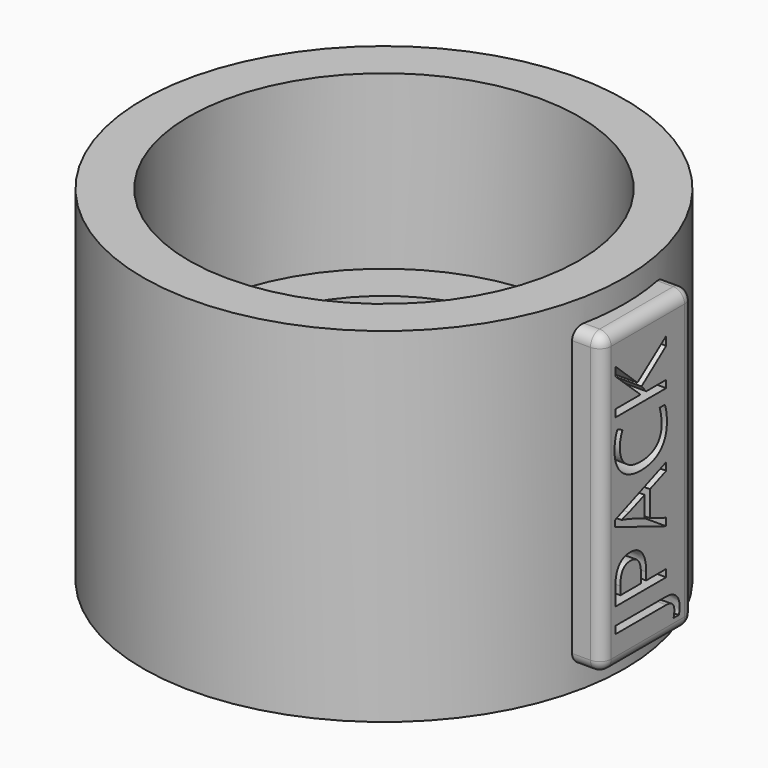
from build123d import *

# Parameters (mm, degrees)
F3_R          = 10.5
F4_DEPTH      = 2
F0_R          = 10.5
F0_R_2        = 6.5
F5_DEPTH      = 5.5
F6_R          = 10.5
F6_R_2        = 8.5
F7_DEPTH      = 7.5
F10_DEPTH     = 2
F11_R         = 0.5
F12_TEXT_SIZE = 3.8888888889
F13_DEPTH     = 5
F14_DEPTH     = 25


# Not quite as in the source:
# - Text() gives the source's letters only with a copy of the font that has no kerning and outlines rounded to 1/6400 em; it was checked with that copy


with BuildPart() as f4:
    # F3 (on offset) → F4 (new body)
    with BuildSketch(Plane.XY.offset(5.5)):
        Circle(F3_R)
    extrude(amount=F4_DEPTH)

    # F0 (on Top) → F5 (join)
    with BuildSketch(Plane.XY):
        Circle(F0_R)
        Circle(F0_R_2, mode=Mode.SUBTRACT)
    extrude(amount=F5_DEPTH)

    # F6 (on offset) → F7 (join)
    with BuildSketch(Plane.XY.offset(7.5)):
        Circle(F6_R)
        Circle(F6_R_2, mode=Mode.SUBTRACT)
    extrude(amount=F7_DEPTH)

    # F9 (on offset) → F10 (join)
    with BuildSketch(Plane.YZ.offset(9.5)):
        Polygon((-2.5, 1), (0, 1), (2.5, 1), (2.5, 14), (0, 14), (-2.5, 14), align=None)
    extrude(amount=F10_DEPTH)

    # F11
    f11_edges = [f4.edges().sort_by_distance(p)[0] for p in [
        (11.5, 0, 14),
        (11.5, 2.5, 7.5),
        (11.5, 0, 1),
        (11.5, -2.5, 7.5),
        (10.84902, 2.5, 14),
        (10.84902, 2.5, 1),
        (10.84902, -2.5, 14),
        (10.84902, -2.5, 1),
    ]]
    fillet(f11_edges, radius=F11_R)

    # F12 (on offset) → F13 (cut)
    with BuildSketch(Plane.YZ.offset(9.5)):
        with Locations(Location((1, 2), (0, 0, 90))):
            Text('JPACK', F12_TEXT_SIZE, font='Open Sans', text_align=(TextAlign.LEFT, TextAlign.BOTTOM))
    extrude(amount=F13_DEPTH, mode=Mode.SUBTRACT)

    # F14 (cut): a face of the model
    f14_faces = [f4.faces().sort_by_distance(p)[0] for p in [
        (0, 0, 5.5),
    ]]
    extrude(f14_faces, amount=-F14_DEPTH, mode=Mode.SUBTRACT)


solid = f4.part
